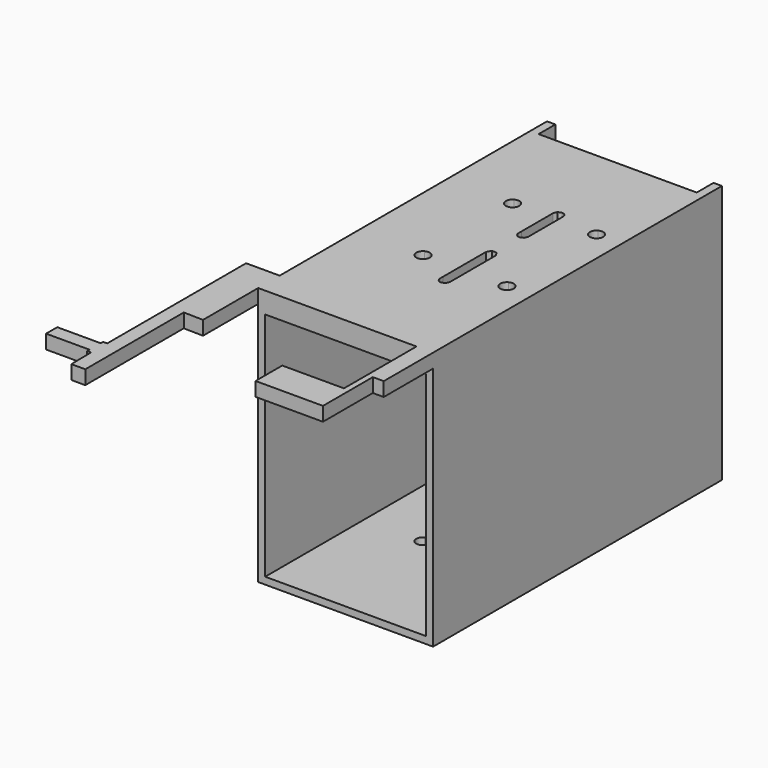
from build123d import *

# Parameters (mm, degrees)
F1_DEPTH = 185
F3_DEPTH = 10
F4_W     = 115
F4_H     = 165
F5_DEPTH = 258.000905792


# Not quite as in the source:
# - ends of sketch curves that miss each other by under 0.0002 mm in the source are joined


with BuildPart() as f1:
    # F0 (on Top) → F1 (new body)
    with BuildSketch(Plane.XY):
        Polygon((-15195.8566048656, 3549.5973710862), (-15195.8566048656, 3439.5974354462), (-15189.8565415216, 3439.5974354462), (-15076.8565772096, 3439.5974354462), (-15070.8566048656, 3439.5974354462), (-15070.8566048656, 3697.5973412382), (-15076.8565772096, 3697.5973412382), (-15076.8565772096, 3682.5973608782), (-15078.8566286576, 3682.5973608782), (-15187.8565810736, 3682.5974354462), (-15189.8565415216, 3682.5973608782), (-15189.8565415216, 3697.5973412382), (-15195.8566048656, 3697.5973412382), (-15195.8566048656, 3585.5973601502), align=None)
        with BuildLine():
            ThreePointArc((-15144.6997061181, 3525.6974171434), (-15147.0197342214, 3523.6627784792), (-15150.0989466253, 3523.4609471966))
            ThreePointArc((-15150.0989466253, 3523.4609471966), (-15153.6155485599, 3527.4708877205), (-15151.2565905183, 3532.2543395114))
            ThreePointArc((-15151.2565905183, 3532.2543395114), (-15148.2300473551, 3532.8563331125), (-15145.4624530362, 3531.4915005715))
            ThreePointArc((-15145.4624530362, 3531.4915005715), (-15144.4219501435, 3529.9342749734), (-15144.0565882627, 3528.0974002701))
            ThreePointArc((-15144.0565882627, 3528.0974002701), (-15144.2201615374, 3526.8550735884), (-15144.6997061181, 3525.6974171434))
        make_face(mode=Mode.SUBTRACT)
        with BuildLine():
            Line((-15116.8566281696, 3553.0971588701), (-15116.8566281696, 3512.0973846862))
            Line((-15116.8566281696, 3512.0973846862), (-15117.8817463992, 3509.6225121318))
            Line((-15117.8817463992, 3509.6225121318), (-15120.3565849536, 3508.5973859022))
            ThreePointArc((-15120.3565849536, 3508.5973859022), (-15121.6959964511, 3508.8638002163), (-15122.831495399, 3509.6225112408))
            ThreePointArc((-15122.831495399, 3509.6225112408), (-15123.5902020342, 3510.7579925208), (-15123.8566267376, 3512.0973846862))
            Line((-15123.8566267376, 3512.0973846862), (-15123.8566257376, 3514.5974072462))
            Line((-15123.8566257376, 3514.5974072462), (-15123.8566257376, 3550.5973973102))
            Line((-15123.8566257376, 3550.5973973102), (-15123.8566257376, 3553.0973698702))
            Line((-15123.8566257376, 3553.0973698702), (-15122.1065173456, 3556.1284925492))
            Line((-15122.1065173456, 3556.1284925492), (-15118.6064755616, 3556.1284075491))
            Line((-15118.6064755616, 3556.1284075491), (-15116.8566281696, 3553.0971588701))
        make_face(mode=Mode.SUBTRACT)
        with BuildLine():
            ThreePointArc((-15084.6996789281, 3525.6974167104), (-15087.0197074586, 3523.6627781987), (-15090.0989201183, 3523.4609474466))
            ThreePointArc((-15090.0989201183, 3523.4609474466), (-15093.6155167933, 3527.4708474467), (-15091.2566211137, 3532.2542928082))
            ThreePointArc((-15091.2566211137, 3532.2542928082), (-15088.2301039392, 3532.8563372409), (-15085.46250991, 3531.4915002578))
            ThreePointArc((-15085.46250991, 3531.4915002578), (-15084.4220063253, 3529.9342687673), (-15084.0566268224, 3528.0973922701))
            ThreePointArc((-15084.0566268224, 3528.0973922701), (-15084.2201743773, 3526.8550755384), (-15084.6996789281, 3525.6974167104))
        make_face(mode=Mode.SUBTRACT)
        with BuildLine():
            ThreePointArc((-15144.0565852624, 3608.0974171902), (-15144.2201528754, 3606.8550614278), (-15144.6997058005, 3605.6973778801))
            ThreePointArc((-15144.6997058005, 3605.6973778801), (-15152.2507291192, 3604.7033006534), (-15151.2566180172, 3612.2543480604))
            ThreePointArc((-15151.2566180172, 3612.2543480604), (-15148.2300485584, 3612.8562968319), (-15145.4624534505, 3611.4914680773))
            ThreePointArc((-15145.4624534505, 3611.4914680773), (-15144.4219579335, 3609.9342657493), (-15144.0565852624, 3608.0974171902))
        make_face(mode=Mode.SUBTRACT)
        with BuildLine():
            Line((-15116.8566281696, 3613.0973553102), (-15116.8566281696, 3582.0973613662))
            Line((-15116.8566281696, 3582.0973613662), (-15117.8817463992, 3579.6225228118))
            Line((-15117.8817463992, 3579.6225228118), (-15120.3565849536, 3578.5974045822))
            ThreePointArc((-15120.3565849536, 3578.5974045822), (-15121.6959954752, 3578.8638152609), (-15122.8314944995, 3579.6225228203))
            ThreePointArc((-15122.8314944995, 3579.6225228203), (-15123.5901954685, 3580.757987549), (-15123.8566257374, 3582.0973613662))
            Line((-15123.8566257374, 3582.0973613662), (-15123.8566257376, 3584.5973769262))
            Line((-15123.8566257376, 3584.5973769262), (-15123.8566257376, 3610.5973817502))
            Line((-15123.8566257376, 3610.5973817502), (-15123.8566257376, 3613.0973553102))
            Line((-15123.8566257376, 3613.0973553102), (-15122.831494508, 3615.5722278646))
            Line((-15122.831494508, 3615.5722278646), (-15120.3565849536, 3616.5973540942))
            ThreePointArc((-15120.3565849536, 3616.5973540942), (-15119.0172109093, 3616.3309267174), (-15117.8817462717, 3615.5722279921))
            ThreePointArc((-15117.8817462717, 3615.5722279921), (-15117.1230451539, 3614.4367462649), (-15116.8566281696, 3613.0973553102))
        make_face(mode=Mode.SUBTRACT)
        with BuildLine():
            ThreePointArc((-15084.6996785285, 3605.6973773998), (-15087.0197077368, 3603.662743742), (-15090.0989201433, 3603.4609502731))
            ThreePointArc((-15090.0989201433, 3603.4609502731), (-15093.6155156943, 3607.4708475063), (-15091.2566491127, 3612.2543022227))
            ThreePointArc((-15091.2566491127, 3612.2543022227), (-15088.2301051425, 3612.8563009603), (-15085.4625103242, 3611.4914677636))
            ThreePointArc((-15085.4625103242, 3611.4914677636), (-15084.4220132506, 3609.9342598695), (-15084.0566228228, 3608.0974091893))
            ThreePointArc((-15084.0566228228, 3608.0974091893), (-15084.2201647807, 3606.855063136), (-15084.6996785285, 3605.6973773998))
        make_face(mode=Mode.SUBTRACT)
    extrude(amount=F1_DEPTH)

    # F2 (on face) → F3 (join)
    with BuildSketch(Plane.XY.offset(185)):
        Polygon((-15253.8564958576, 3322.5974582382), (-15222.8565019136, 3322.5974582382), (-15222.8565019136, 3320.5165420655), (-15220.0527313578, 3320.5165420655), (-15219.8565162416, 3302.6135837618), (-15209.8566090016, 3302.6135837618), (-15209.8566090016, 3390.5974254702), (-15195.8566048656, 3390.3064727783), (-15195.8566048656, 3458.779335022), (-15219.8565162416, 3458.779335022), (-15219.8565162416, 3334.7086508815), (-15222.8565019136, 3334.7086508815), (-15222.8565019136, 3332.5974504782), (-15253.8564958576, 3332.5974504782), align=None)
        Polygon((-15070.8566048656, 3395.4774719814), (-15070.8566048656, 3439.5974354462), (-15082.7350530551, 3439.5974354462), (-15082.7350530551, 3374.8135232611), (-15126.8566124096, 3374.8135232611), (-15126.8566124096, 3350.95351759), (-15078.6617271557, 3350.95351759), (-15078.6617271557, 3395.4774719814), align=None)
    extrude(amount=-F3_DEPTH)

    # F4 (on face) → F5 (cut, through all)
    with BuildSketch(Plane.XZ.offset(-3439.5974354462)):
        with Locations((-15133.3566048656, 87.5)):
            Rectangle(F4_W, F4_H)
    extrude(amount=-F5_DEPTH, mode=Mode.SUBTRACT)


solid = f1.part
